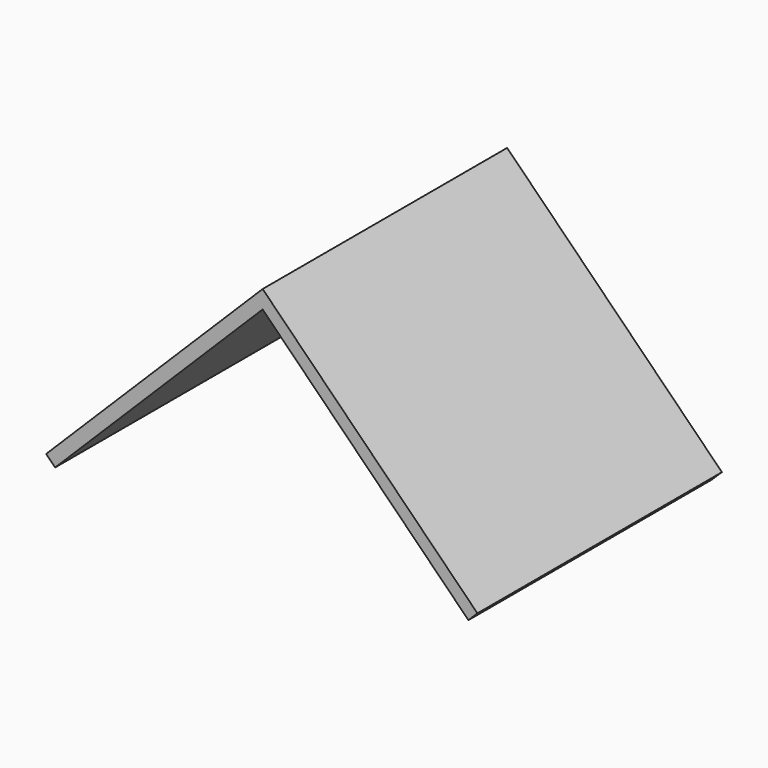
from build123d import *

# Parameters (mm, degrees)
F1_DEPTH     = 1219.2
F3_DEPTH     = 5.08
F4_TEXT_SIZE = 311.9106376821
F5_DEPTH     = 25.4


# Not quite as in the source:
# - Text() gives the source's letters only with a copy of the font that has no kerning and outlines rounded to 1/6400 em; it was checked with that copy


with BuildPart() as f1:
    # F0 (on Front) → F1 (new body)
    with BuildSketch(Plane.XZ):
        Polygon((860.3227629429, 0), (0, 863.8827371595), (-867.4574423782, 0), (-831.1638198968, -35.8467817893), (0, 791.8918952712), (824.3276488946, -35.8467817893), align=None)
    extrude(amount=F1_DEPTH)

    # F2 (on face) → F3 (join)
    with BuildSketch(Plane(origin=(0, 0, 0), x_dir=(-1, 0, 0), z_dir=(0, 1, 0))):
        Polygon((867.4574423782, 0), (0, 863.8827371595), (-860.3227629429, 0), align=None)
    extrude(amount=F3_DEPTH)

    # F4 (on face) → F5 (cut)
    with BuildSketch(Plane(origin=(0, 5.08, 0), x_dir=(-1, 0, 0), z_dir=(0, 1, 0))):
        with Locations((-441.7357338376, 195.7434629691)):
            Text('Rusty', F4_TEXT_SIZE, font='Open Sans', font_style=FontStyle.BOLD, text_align=(TextAlign.LEFT, TextAlign.BOTTOM))
    extrude(amount=-F5_DEPTH, mode=Mode.SUBTRACT)


solid = f1.part
